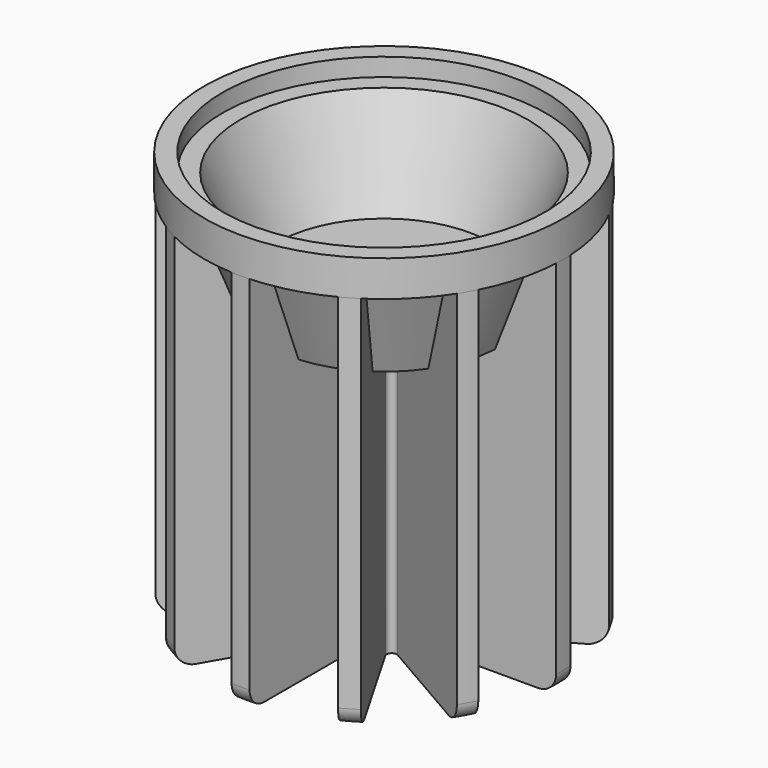
from build123d import *

# Parameters (mm, degrees)
F5_R = 3


# Not quite as in the source:
# - after a boolean that leaves OpenCascade's solid faulty, fix() repairs it


with BuildPart() as f1:
    # F0 (on Right) → F1 (revolve)
    with BuildSketch(Plane.YZ):
        Polygon((-19.7913602038, -12.5343254842), (0, -12.5343254842), (0, -9.5343254842), (-17.7432774566, -9.5343254842), (-24, 6.4656745158), (-27, 6.4656745158), (-27, 9.4656745158), (-30, 9.4656745158), (-30, 3.4656745158), (-26.0480827472, 3.4656745158), align=None)
    revolve(axis=Axis((0, 0, -11.0343254842), (0, 0, -1)))

    # F3 (on offset) → F4 (join, up to the next surface of F1)
    with BuildSketch(Plane.XY.offset(-60)):
        with BuildLine():
            Line((-13.6822001609, -26.698265838), (-3.0822316874, -8.3385818833))
            ThreePointArc((-3.0822316874, -8.3385818833), (-2.1284587501, -7.9435161973), (-1.5, -8.7625395862))
            Line((-1.5, -8.7625395862), (-1.5, -29.9624765332))
            ThreePointArc((-1.5, -29.9624765332), (0, -30), (1.5, -29.9624765332))
            Line((1.5, -29.9624765332), (1.5, -8.7625395862))
            ThreePointArc((1.5, -8.7625395862), (2.1284587501, -7.9435161973), (3.0822316874, -8.3385818833))
            Line((3.0822316874, -8.3385818833), (13.6822001609, -26.698265838))
            ThreePointArc((13.6822001609, -26.698265838), (15, -25.9807621135), (16.2802763723, -25.198265838))
            Line((16.2802763723, -25.198265838), (5.6803078988, -6.8385818833))
            ThreePointArc((5.6803078988, -6.8385818833), (5.8150574471, -5.8150574471), (6.8385818833, -5.6803078988))
            Line((6.8385818833, -5.6803078988), (25.198265838, -16.2802763723))
            ThreePointArc((25.198265838, -16.2802763723), (25.9807621135, -15), (26.698265838, -13.6822001609))
            Line((26.698265838, -13.6822001609), (8.3385818833, -3.0822316874))
            ThreePointArc((8.3385818833, -3.0822316874), (7.9435161973, -2.1284587501), (8.7625395862, -1.5))
            Line((8.7625395862, -1.5), (29.9624765332, -1.5))
            ThreePointArc((29.9624765332, -1.5), (30, 0), (29.9624765332, 1.5))
            Line((29.9624765332, 1.5), (8.7625395862, 1.5))
            ThreePointArc((8.7625395862, 1.5), (7.9435161973, 2.1284587501), (8.3385818833, 3.0822316874))
            Line((8.3385818833, 3.0822316874), (26.698265838, 13.6822001609))
            ThreePointArc((26.698265838, 13.6822001609), (25.9807621135, 15), (25.198265838, 16.2802763723))
            Line((25.198265838, 16.2802763723), (6.8385818833, 5.6803078988))
            ThreePointArc((6.8385818833, 5.6803078988), (5.8150574471, 5.8150574471), (5.6803078988, 6.8385818833))
            Line((5.6803078988, 6.8385818833), (16.2802763723, 25.198265838))
            ThreePointArc((16.2802763723, 25.198265838), (15, 25.9807621135), (13.6822001609, 26.698265838))
            Line((13.6822001609, 26.698265838), (3.0822316874, 8.3385818833))
            ThreePointArc((3.0822316874, 8.3385818833), (2.1284587501, 7.9435161973), (1.5, 8.7625395862))
            Line((1.5, 8.7625395862), (1.5, 29.9624765332))
            ThreePointArc((1.5, 29.9624765332), (0, 30), (-1.5, 29.9624765332))
            Line((-1.5, 29.9624765332), (-1.5, 8.7625395862))
            ThreePointArc((-1.5, 8.7625395862), (-2.1284587501, 7.9435161973), (-3.0822316874, 8.3385818833))
            Line((-3.0822316874, 8.3385818833), (-13.6822001609, 26.698265838))
            ThreePointArc((-13.6822001609, 26.698265838), (-15, 25.9807621135), (-16.2802763723, 25.198265838))
            Line((-16.2802763723, 25.198265838), (-5.6803078988, 6.8385818833))
            ThreePointArc((-5.6803078988, 6.8385818833), (-5.8150574471, 5.8150574471), (-6.8385818833, 5.6803078988))
            Line((-6.8385818833, 5.6803078988), (-25.198265838, 16.2802763723))
            ThreePointArc((-25.198265838, 16.2802763723), (-25.9807621135, 15), (-26.698265838, 13.6822001609))
            Line((-26.698265838, 13.6822001609), (-8.3385818833, 3.0822316874))
            ThreePointArc((-8.3385818833, 3.0822316874), (-7.9435161973, 2.1284587501), (-8.7625395862, 1.5))
            Line((-8.7625395862, 1.5), (-29.9624765332, 1.5))
            ThreePointArc((-29.9624765332, 1.5), (-30, 0), (-29.9624765332, -1.5))
            Line((-29.9624765332, -1.5), (-8.7625395862, -1.5))
            ThreePointArc((-8.7625395862, -1.5), (-7.9435161973, -2.1284587501), (-8.3385818833, -3.0822316874))
            Line((-8.3385818833, -3.0822316874), (-26.698265838, -13.6822001609))
            ThreePointArc((-26.698265838, -13.6822001609), (-25.9807621135, -15), (-25.198265838, -16.2802763723))
            Line((-25.198265838, -16.2802763723), (-6.8385818833, -5.6803078988))
            ThreePointArc((-6.8385818833, -5.6803078988), (-5.8150574471, -5.8150574471), (-5.6803078988, -6.8385818833))
            Line((-5.6803078988, -6.8385818833), (-16.2802763723, -25.198265838))
            ThreePointArc((-16.2802763723, -25.198265838), (-15, -25.9807621135), (-13.6822001609, -26.698265838))
        make_face()
    extrude(until=Until.NEXT)

    add(f1.part.fix(), mode=Mode.REPLACE)

    # F5
    f5_edges = [f1.edges().sort_by_distance(p)[0] for p in [
        (-15, -25.980762, -60),
        (-25.980762, -15, -60),
        (-30, 0, -60),
        (-25.980762, 15, -60),
        (-15, 25.980762, -60),
        (0, 30, -60),
        (15, 25.980762, -60),
        (25.980762, 15, -60),
        (30, 0, -60),
        (25.980762, -15, -60),
        (15, -25.980762, -60),
        (0, -30, -60),
    ]]
    fillet(f5_edges, radius=F5_R)


solid = f1.part
